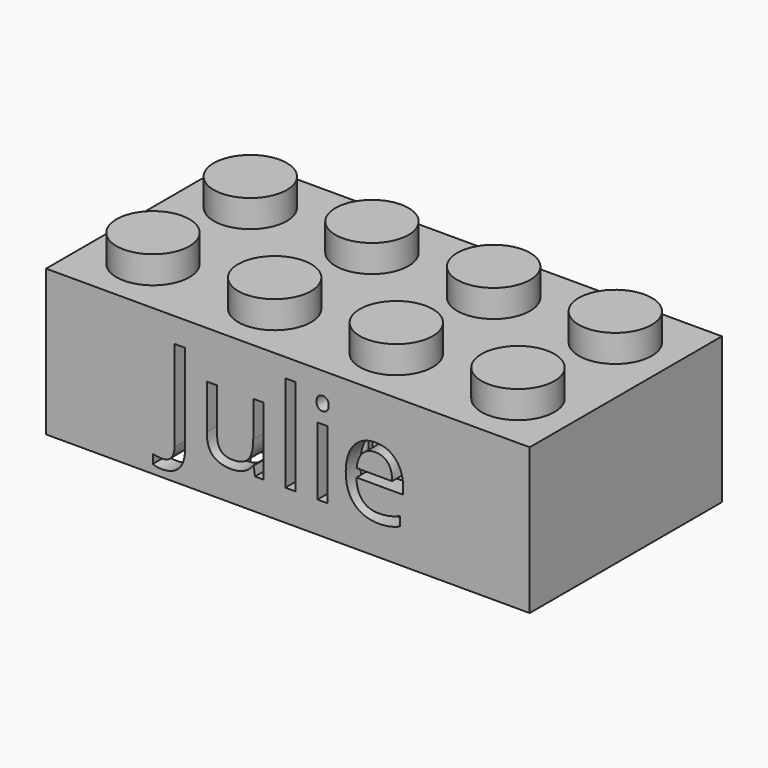
from build123d import *

# Parameters (mm, degrees)
F0_W          = 31.8
F0_H          = 15.8
F1_DEPTH      = 9.6
F2_W          = 29.4
F2_H          = 13.4
F3_DEPTH      = 8.4
F4_R          = 2.4
F5_DEPTH      = 1.8
F6_R          = 1.3
F7_DEPTH      = 1.2
F8_R          = 3.255
F8_R_2        = 2.4
F9_DEPTH      = 8.4
F10_W         = 0.6
F10_H         = 0.3
F11_DEPTH     = 8.4
F12_W         = 0.3
F12_H         = 0.6
F13_DEPTH     = 8.4
F15_W         = 0.6
F15_H         = 4
F15_H_2       = 4.0198345669
F16_DEPTH     = 6.4
F17_TEXT_SIZE = 8.3410213443
F18_DEPTH     = 1.2


# Not quite as in the source:
# - Text() gives the source's letters only with a copy of the font that has no kerning and outlines rounded to 1/6400 em; it was checked with that copy


with BuildPart() as f1:
    # F0 (on Top) → F1 (new body)
    with BuildSketch(Plane.XY):
        Rectangle(F0_W, F0_H)
    extrude(amount=F1_DEPTH)

    # F2 (on face) → F3 (cut)
    with BuildSketch(Plane(origin=(0, 0, 0), x_dir=(1, 0, 0), z_dir=(0, 0, -1))):
        Rectangle(F2_W, F2_H)
    extrude(amount=-F3_DEPTH, mode=Mode.SUBTRACT)

    # F4 (on face) → F5 (join)
    with BuildSketch(Plane.XY.offset(9.6)):
        with Locations((-11.95, 3.95)):
            Circle(F4_R)
        with Locations((-3.95, 3.95)):
            Circle(F4_R)
        with Locations((4.05, 3.95)):
            Circle(F4_R)
        with Locations((12.05, 3.95)):
            Circle(F4_R)
        with Locations((-11.95, -4.05)):
            Circle(F4_R)
        with Locations((-3.95, -4.05)):
            Circle(F4_R)
        with Locations((4.05, -4.05)):
            Circle(F4_R)
        with Locations((12.05, -4.05)):
            Circle(F4_R)
    extrude(amount=F5_DEPTH)

    # F6 (on face) → F7 (cut)
    with BuildSketch(Plane(origin=(0, 0, 8.4), x_dir=(1, 0, 0), z_dir=(0, 0, -1))):
        with Locations((-11.95, 3.95)):
            Circle(F6_R)
        with Locations((-11.95, -4.05)):
            Circle(F6_R)
        with Locations((-3.95, 3.95)):
            Circle(F6_R)
        with Locations((-3.95, -4.05)):
            Circle(F6_R)
        with Locations((4.05, 3.95)):
            Circle(F6_R)
        with Locations((4.05, -4.05)):
            Circle(F6_R)
        with Locations((12.05, 3.95)):
            Circle(F6_R)
        with Locations((12.05, -4.05)):
            Circle(F6_R)
    extrude(amount=-F7_DEPTH, mode=Mode.SUBTRACT)

    # F8 (on face) → F9 (join, through all)
    with BuildSketch(Plane(origin=(0, 0, 8.4), x_dir=(1, 0, 0), z_dir=(0, 0, -1))):
        with Locations((-7.95, -0.05)):
            Circle(F8_R)
        with Locations((-7.95, -0.05)):
            Circle(F8_R_2, mode=Mode.SUBTRACT)
        with Locations((0.05, -0.05)):
            Circle(F8_R)
        with Locations((0.05, -0.05)):
            Circle(F8_R_2, mode=Mode.SUBTRACT)
        with Locations((8.05, -0.05)):
            Circle(F8_R)
        with Locations((8.05, -0.05)):
            Circle(F8_R_2, mode=Mode.SUBTRACT)
    extrude(amount=F9_DEPTH)

    # F10 (on face) → F11 (join, through all)
    with BuildSketch(Plane(origin=(0, 0, 0), x_dir=(1, 0, 0), z_dir=(0, 0, -1))):
        with Locations((-11.95, 6.55)):
            Rectangle(F10_W, F10_H)
        with Locations((-11.95, -6.55)):
            Rectangle(F10_W, F10_H)
        with Locations((-3.95, 6.55)):
            Rectangle(F10_W, F10_H)
        with Locations((-3.95, -6.55)):
            Rectangle(F10_W, F10_H)
        with Locations((4.05, 6.55)):
            Rectangle(F10_W, F10_H)
        with Locations((4.05, -6.55)):
            Rectangle(F10_W, F10_H)
        with Locations((12.05, 6.55)):
            Rectangle(F10_W, F10_H)
        with Locations((12.05, -6.55)):
            Rectangle(F10_W, F10_H)
    extrude(amount=-F11_DEPTH)

    # F12 (on face) → F13 (join, through all)
    with BuildSketch(Plane(origin=(0, 0, 0), x_dir=(1, 0, 0), z_dir=(0, 0, -1))):
        with Locations((-14.55, 4.05)):
            Rectangle(F12_W, F12_H)
        with Locations((-14.55, -3.95)):
            Rectangle(F12_W, F12_H)
        with Locations((14.55, 4.05)):
            Rectangle(F12_W, F12_H)
        with Locations((14.55, -3.95)):
            Rectangle(F12_W, F12_H)
    extrude(amount=-F13_DEPTH)

    # F15 (on offset) → F16 (join)
    with BuildSketch(Plane.XY.offset(8.4)):
        with Locations((0, -4.9997619353)):
            Rectangle(F15_W, F15_H)
        with Locations((0, 4.9143608194)):
            Rectangle(F15_W, F15_H_2)
    extrude(amount=-F16_DEPTH)

    # F17 (on face) → F18 (cut)
    with BuildSketch(Plane.XZ.offset(7.9)):
        with Locations((-8.2308937968, 2.0341328345)):
            Text('Julie', F17_TEXT_SIZE, font='Open Sans', text_align=(TextAlign.LEFT, TextAlign.BOTTOM))
    extrude(amount=-F18_DEPTH, mode=Mode.SUBTRACT)


solid = f1.part
